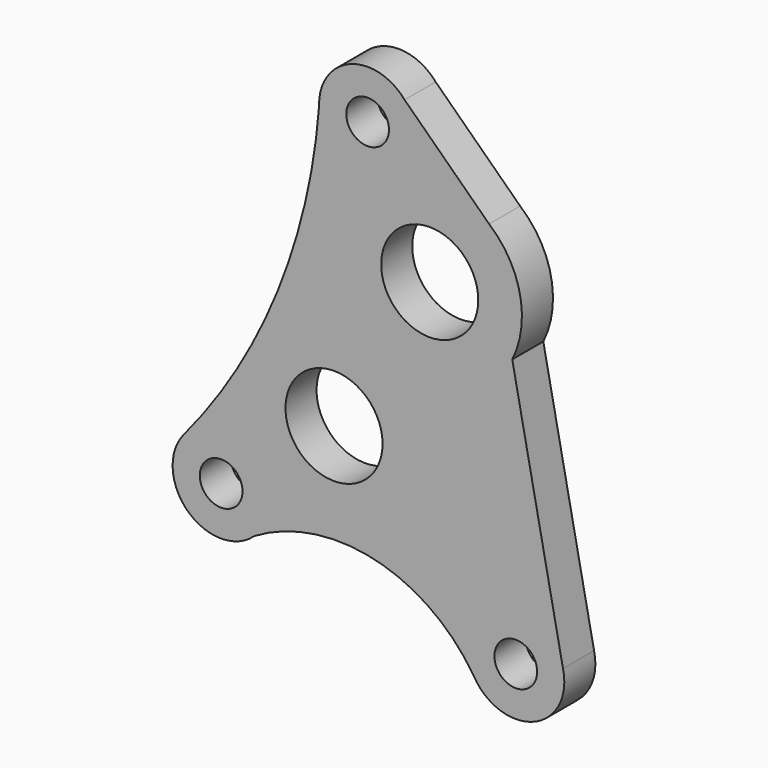
from build123d import *

# Parameters (mm, degrees)
F0_R     = 4.4
F0_R_2   = 10
F1_DEPTH = 8


# Not quite as in the source:
# - a feature names something its author has since deleted; it is built from what else it names


with BuildPart() as f1:
    # F0 (on Front) → F1 (new body)
    with BuildSketch(Plane.XZ):
        with BuildLine():
            Line((31.9492522213, 47.021704051), (14.5416913837, 63.871923339))
            ThreePointArc((14.5416913837, 63.871923339), (3.3211707837, 66.7258087658), (-3.0733272697, 57.0741177632))
            ThreePointArc((-3.0733272697, 57.0741177632), (-11.6409365793, 20.6574209247), (-30.8284920773, -11.4582676391))
            ThreePointArc((-30.8284920773, -11.4582676391), (-30.197435382, -25.1853746986), (-16.4565083148, -25.3218448705))
            ThreePointArc((-16.4565083148, -25.3218448705), (8.288194067, -21.4806704364), (28.7486613668, -35.9175743588))
            ThreePointArc((28.7486613668, -35.9175743588), (41.111240011, -40.2846954641), (47.1716852414, -28.6581697108))
            Line((47.1716852414, -28.6581697108), (36.7147233028, 24.0100747195))
            ThreePointArc((36.7147233028, 24.0100747195), (38.3163132105, 36.3410020894), (31.9492522213, 47.021704051))
        make_face()
        with Locations((-23.2548138211, -17.9881526052)):
            Circle(F0_R, mode=Mode.SUBTRACT)
        Circle(F0_R_2, mode=Mode.SUBTRACT)
        with Locations((37.4451861789, -30.9809301349)):
            Circle(F0_R, mode=Mode.SUBTRACT)
        with Locations((6.9214779515, 57.3964042673)):
            Circle(F0_R, mode=Mode.SUBTRACT)
        with Locations((19.7110784827, 32.4880498807)):
            Circle(F0_R_2, mode=Mode.SUBTRACT)
    extrude(amount=F1_DEPTH)


solid = f1.part
